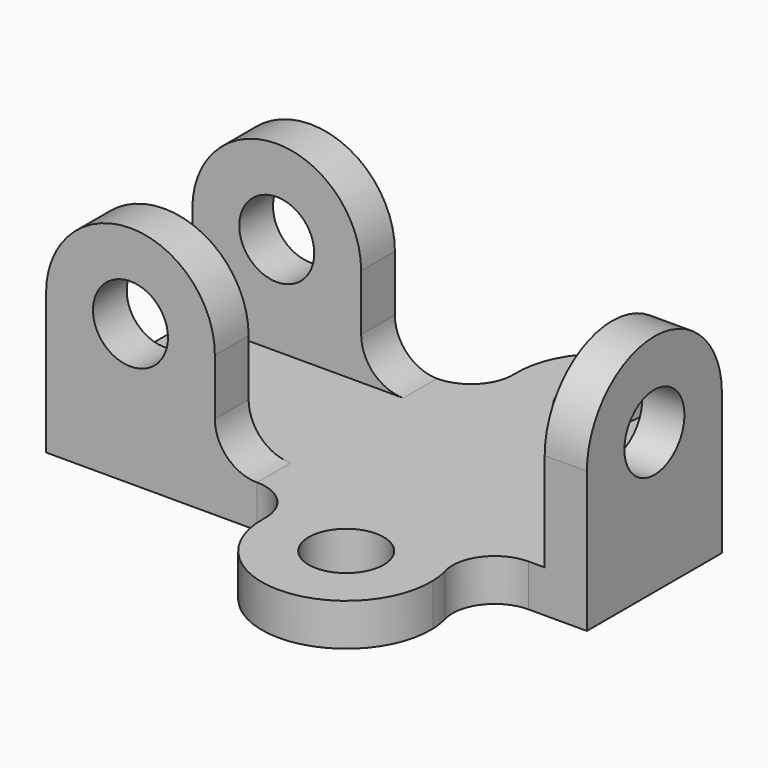
from build123d import *

# Parameters (mm, degrees)
F0_R     = 8
F1_DEPTH = 9
F3_DEPTH = 9
F4_R     = 8
F5_DEPTH = 9
F7_DEPTH = 9
F8_R     = 8
F9_DEPTH = 9


# Not quite as in the source:
# - a pattern or mirror of a feature is missing from the dataset's text; its kind, count and spacing are read off the source's solid


with BuildPart() as f1:
    # F0 (on Top) → F1 (new body)
    with BuildSketch(Plane.XY):
        with BuildLine():
            ThreePointArc((17.3845397472, 29.3333333333), (17.7988188757, 31.316337087), (17.9876500843, 33.3333333333))
            ThreePointArc((17.9876500843, 33.3333333333), (0, 52), (-17.9876500843, 33.3333333333))
            ThreePointArc((-17.9876500843, 33.3333333333), (-20.5007344281, 26.7550020016), (-26.9814751265, 24))
            Line((-26.9814751265, 24), (-72, 24))
            Line((-72, 24), (-72, -24))
            Line((-72, -24), (-26.9814751265, -24))
            ThreePointArc((-26.9814751265, -24), (-20.5007344281, -26.7550020016), (-17.9876500843, -33.3333333333))
            ThreePointArc((-17.9876500843, -33.3333333333), (0, -52), (17.9876500843, -33.3333333333))
            ThreePointArc((17.9876500843, -33.3333333333), (17.7988188757, -31.316337087), (17.3845397472, -29.3333333333))
            ThreePointArc((17.3845397472, -29.3333333333), (18.9353811923, -21.5227744249), (26.0768096208, -18))
            Line((26.0768096208, -18), (38.5327786207, -18))
            Line((38.5327786207, -18), (38.5327786207, 18))
            Line((38.5327786207, 18), (26.0768096208, 18))
            ThreePointArc((26.0768096208, 18), (18.9353811923, 21.5227744249), (17.3845397472, 29.3333333333))
        make_face()
        with Locations((0, -34)):
            Circle(F0_R, mode=Mode.SUBTRACT)
        with Locations((0, 34)):
            Circle(F0_R, mode=Mode.SUBTRACT)
    extrude(amount=F1_DEPTH)

    # F2 (on face) → F3 (join)
    with BuildSketch(Plane.XZ.offset(24)):
        with BuildLine():
            Line((-36.0185248735, 18), (-36.0185248735, 30))
            ThreePointArc((-36.0185248735, 30), (-54.0264671065, 47.9999982478), (-72.0185178648, 29.9841155356))
            Line((-72.0185178648, 29.9841155356), (-72, 9))
            Line((-72, 9), (-27.0185248735, 9))
            ThreePointArc((-27.0185248735, 9), (-33.3824859042, 11.6360389693), (-36.0185248735, 18))
        make_face()
    f3 = extrude(amount=-F3_DEPTH)

    # F3_copies: F3 across plane
    add(f3.mirror(Plane.ZX))

    # F4 (on face) → F5 (cut, through all)
    with BuildSketch(Plane.XZ.offset(24)):
        with Locations((-54.0185248735, 30)):
            Circle(F4_R)
    f5 = extrude(amount=-F5_DEPTH, mode=Mode.SUBTRACT)

    # F5_copies: F5 across plane
    add(f5.mirror(Plane.ZX), mode=Mode.SUBTRACT)

    # F6 (on face) → F7 (join)
    with BuildSketch(Plane.YZ.offset(38.5327786207)):
        with BuildLine():
            Line((18, 9), (18, 30))
            ThreePointArc((18, 30), (0, 48), (-18, 30))
            Line((-18, 30), (-18, 9))
            Line((-18, 9), (18, 9))
        make_face()
    extrude(amount=-F7_DEPTH)

    # F8 (on face) → F9 (cut, through all)
    with BuildSketch(Plane.YZ.offset(38.5327786207)):
        with Locations((0, 30)):
            Circle(F8_R)
    extrude(amount=-F9_DEPTH, mode=Mode.SUBTRACT)


solid = f1.part
